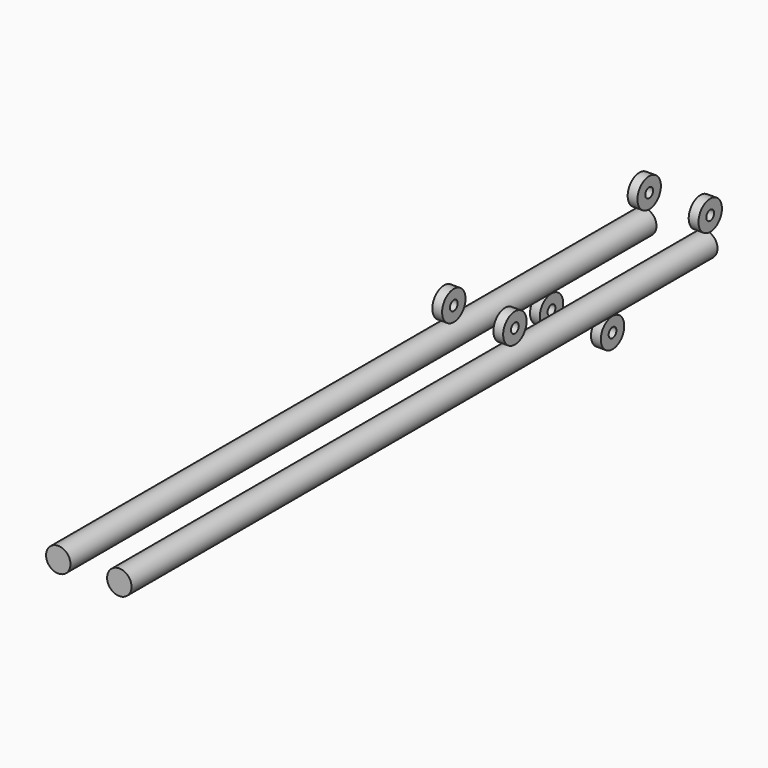
from build123d import *

# Parameters (mm, degrees)
F3_R      = 5
F4_DEPTH  = 300
F9_R      = 6
F9_R_2    = 2
F10_DEPTH = 2


with BuildPart() as f4:
    # F3 (on Front) → F4 (new body)
    with BuildSketch(Plane.XZ):
        Circle(F3_R)
    extrude(amount=F4_DEPTH)


with BuildPart() as f4_1:
    # F5: moved
    add(f4.part.moved(Location((-50, 0, 0))))


with BuildPart() as f10:
    # F9 (on Right) → F10 (new body, symmetric)
    with BuildSketch(Plane.YZ):
        Circle(F9_R)
        Circle(F9_R_2, mode=Mode.SUBTRACT)
    extrude(amount=F10_DEPTH, both=True)


with BuildPart() as f10_1:
    # F11: moved
    add(f10.part.moved(Location((-50, 0, 11))))


with BuildPart() as f12_1:
    # F12: copy of F10
    add(f10_1.part.moved(Location((0, -100, 0))))


with BuildPart() as f13_1:
    # F13: copy of F10
    add(f10_1.part.moved(Location((0, -50, -22))))


with BuildPart() as f14_1:
    # F14: copy of F4
    add(f4_1.part.moved(Location((25, 0, 0))))


with BuildPart() as f14_2:
    # F14: copy of F10
    add(f10_1.part.moved(Location((25, 0, 0))))


with BuildPart() as f14_3:
    # F14: copy of F12_1
    add(f12_1.part.moved(Location((25, 0, 0))))


with BuildPart() as f14_4:
    # F14: copy of F13_1
    add(f13_1.part.moved(Location((25, 0, 0))))


solid = Compound([f4_1.part, f10_1.part, f12_1.part, f13_1.part, f14_1.part, f14_2.part, f14_3.part, f14_4.part])
